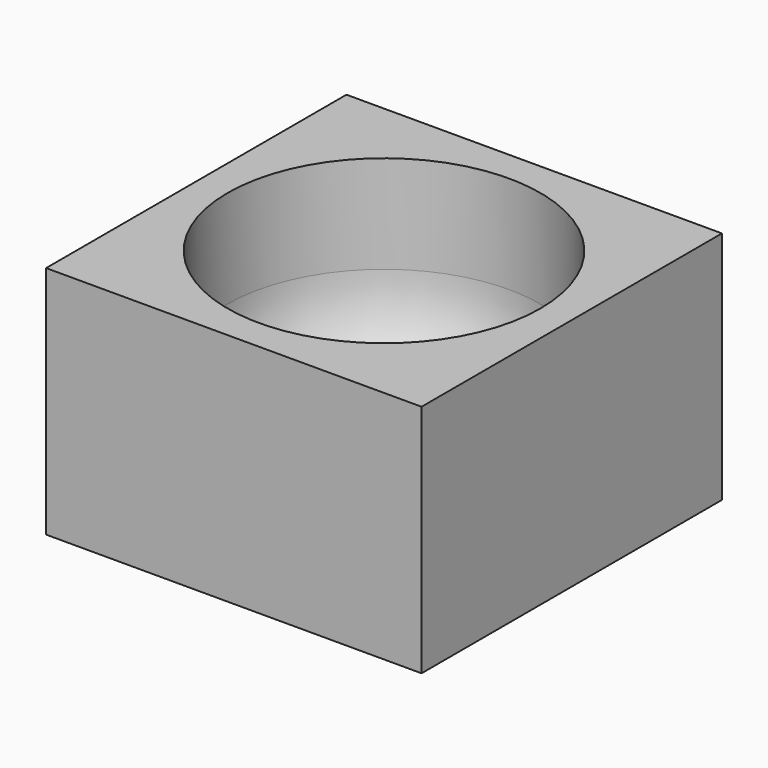
from build123d import *

# Parameters (mm, degrees)
F0_W         = 121.92
F0_H         = 121.92
F1_DEPTH     = 76.2
F2_R         = 50.8
F3_DEPTH     = 69.85
F4_R         = 38.1
F5_TEXT_SIZE = 50.0052733345
F6_DEPTH     = 3.81


# Not quite as in the source:
# - Text() gives the source's letters only with a copy of the font that has no kerning and outlines rounded to 1/6400 em; it was checked with that copy


with BuildPart() as f1:
    # F0 (on Top) → F1 (new body)
    with BuildSketch(Plane.XY):
        Rectangle(F0_W, F0_H)
    extrude(amount=F1_DEPTH)

    # F2 (on face) → F3 (cut)
    with BuildSketch(Plane.XY.offset(76.2)):
        Circle(F2_R)
    extrude(amount=-F3_DEPTH, mode=Mode.SUBTRACT)

    # F4
    f4_edges = [f1.edges().sort_by_distance(p)[0] for p in [
        (-50.8, 0, 6.35),
    ]]
    fillet(f4_edges, radius=F4_R)

    # F5 (on face) → F6 (cut)
    with BuildSketch(Plane(origin=(-60.96, 0, 0), x_dir=(0, -1, 0), z_dir=(-1, 0, 0))):
        with Locations((-44.5372493269, 21.072268183)):
            Text('Ella', F5_TEXT_SIZE, font='Open Sans', font_style=FontStyle.BOLDITALIC, text_align=(TextAlign.LEFT, TextAlign.BOTTOM))
    extrude(amount=-F6_DEPTH, mode=Mode.SUBTRACT)


solid = f1.part
